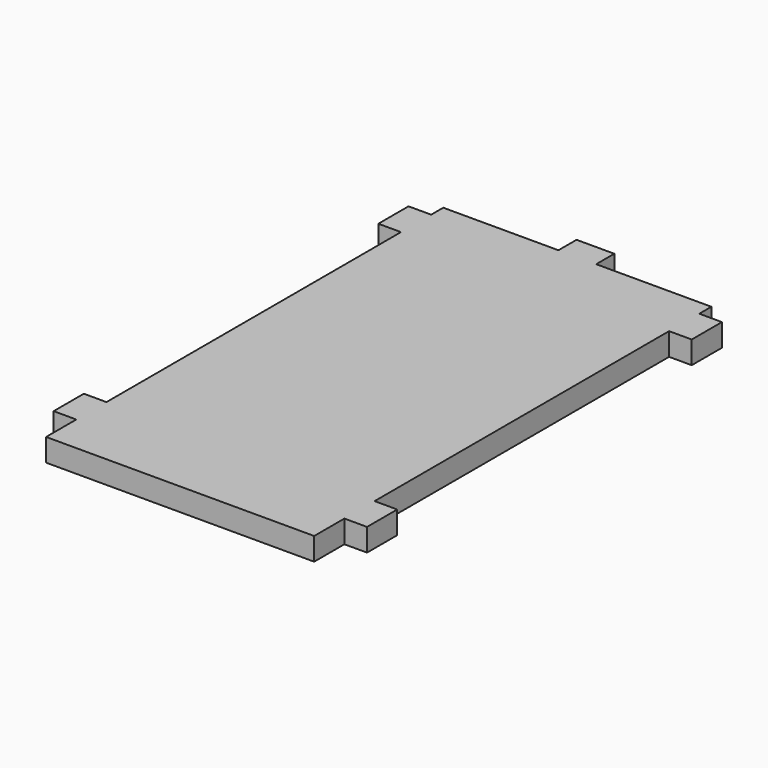
from build123d import *

# Parameters (mm, degrees)
F0_W     = 12
F0_H     = 20
F1_DEPTH = 12


# Not quite as in the source:
# - a feature names something its author has since deleted; it is built from what else it names


with BuildPart() as f1:
    # F0 (on Top) → F1 (new body)
    with BuildSketch(Plane.XY):
        with Locations((-77.025, 107.52248)):
            Rectangle(F0_W, F0_H)
        Polygon((71.025, 125.52248), (10, 125.52248), (-10, 125.52248), (-71.025, 125.52248), (-71.025, 117.52248), (-71.025, 97.52248), (-71.025, -97.52248), (-71.025, -117.52248), (-71.025, -137.52248), (71.025, -137.52248), (71.025, -117.52248), (71.025, -97.52248), (71.025, 97.52248), (71.025, 117.52248), align=None)
        with Locations((77.025, 107.52248)):
            Rectangle(F0_W, F0_H)
        with Locations((-77.025, -107.52248)):
            Rectangle(F0_W, F0_H)
        with Locations((77.025, -107.52248)):
            Rectangle(F0_W, F0_H)
        Polygon((10, 127.52248), (10, 137.52248), (-10, 137.52248), (-10, 127.52248), (-10, 125.52248), (10, 125.52248), align=None)
    extrude(amount=F1_DEPTH)


solid = f1.part
